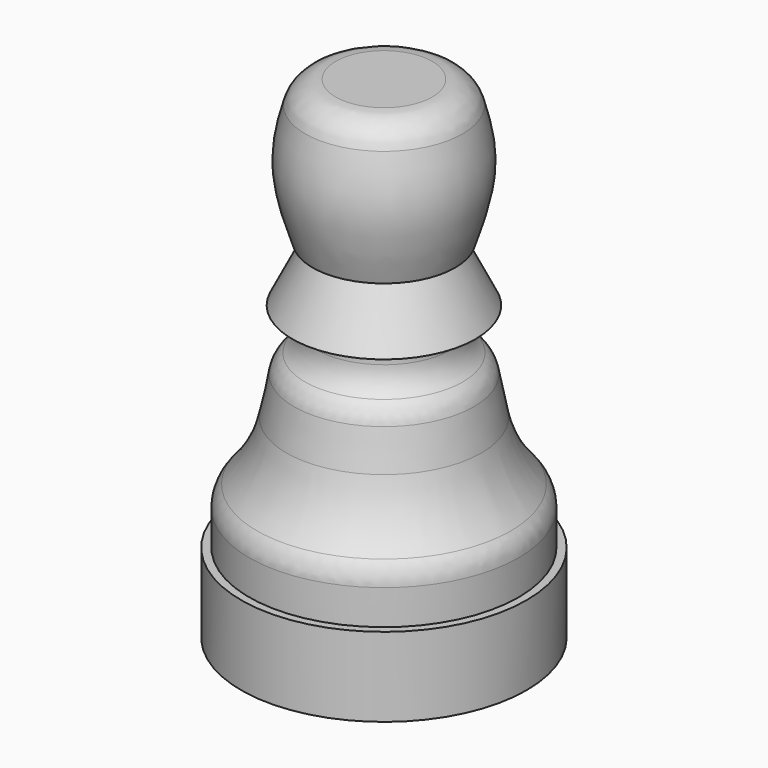
from build123d import *

# Parameters (mm, degrees)
F4_R = 2
F5_R = 2
F6_R = 2


# Not quite as in the source:
# - a fillet or chamfer that OpenCascade refuses, or shapes differently, is made with other operations: its cross-section is extruded or revolved along the edge and cut away or added


with BuildPart() as f1:
    # F0 (on Front) → F1 (revolve)
    with BuildSketch(Plane.XZ):
        with BuildLine():
            Line((0, 31), (0, 0))
            Line((0, 0), (9, 0))
            Line((9, 0), (9, 5))
            Line((9, 5), (8.5, 5))
            Line((8.5, 5), (8.5, 8))
            Line((8.5, 8), (7, 8))
            Line((7, 8), (5.5, 15.5))
            Line((5.5, 15.5), (4.25, 15.5))
            Line((4.25, 15.5), (4.25, 18))
            Line((4.25, 18), (6, 18))
            Line((6, 18), (4, 22))
            Line((4, 22), (4.5, 22))
            add(Edge.make_bspline(
                [(4.5, 31), (5, 29.5), (6, 26.5), (5, 23.5), (4.5, 22)],
                knots=[0, 0, 0, 0, 0.5, 1, 1, 1, 1], degree=3))
            Line((4.5, 31), (0, 31))
        make_face()
    revolve(axis=Axis((0, 0, 15.5), (0, 0, 1)))

    # F2: fillet of radius 2 on 1 edges, made by hand

    # F2_s1 → F2_t2 (revolve)
    with BuildSketch(Plane.XZ):
        with BuildLine():
            ThreePointArc((5.5, 15.5), (4.5916876048, 16.236015633), (4.25, 17.3540496218))
            Line((4.25, 17.3540496218), (4.25, 15.5))
            Line((4.25, 15.5), (5.5, 15.5))
        make_face()
    revolve(axis=Axis((0, 0, 15.5), (0, 0, 1)))

    # F3: fillet of radius 8 on 1 edges, made by hand

    # F3_s1 → F3_t2 (revolve)
    with BuildSketch(Plane.XZ):
        with BuildLine():
            ThreePointArc((8.5, 8), (6.9960478639, 9.9399549841), (6.1510825053, 12.2445874734))
            Line((6.1510825053, 12.2445874734), (5.9941895972, 12.2132088918))
            Line((5.9941895972, 12.2132088918), (6.8431070919, 7.9686214184))
            Line((6.8431070919, 7.9686214184), (7, 7.84))
            ThreePointArc((7, 7.84), (7.75, 7.84), (8.3900854418, 7.8837296689))
            Line((8.3900854418, 7.8837296689), (8.5, 8))
        make_face()
    revolve(axis=Axis((0, 0, 8), (0, 0, 1)))

    # F4
    f4_edges = [f1.edges().sort_by_distance(p)[0] for p in [
        (-5.5, 0, 15.5),
    ]]
    fillet(f4_edges, radius=F4_R)

    # F5
    f5_edges = [f1.edges().sort_by_distance(p)[0] for p in [
        (-8.5, 0, 8),
    ]]
    fillet(f5_edges, radius=F5_R)

    # F6
    f6_edges = [f1.edges().sort_by_distance(p)[0] for p in [
        (-4.5, 0, 31),
    ]]
    fillet(f6_edges, radius=F6_R)

    # F7: chamfer of 1.5 x 0.5 on 1 edges, made by hand

    # F7_s1 → F7_t2 (revolve, cut)
    with BuildSketch(Plane.XZ):
        Polygon((5.7763932023, 18.4472135955), (4.5, 18), (6, 18), align=None)
    revolve(axis=Axis((0, 0, 18), (0, 0, 1)), mode=Mode.SUBTRACT)


solid = f1.part
